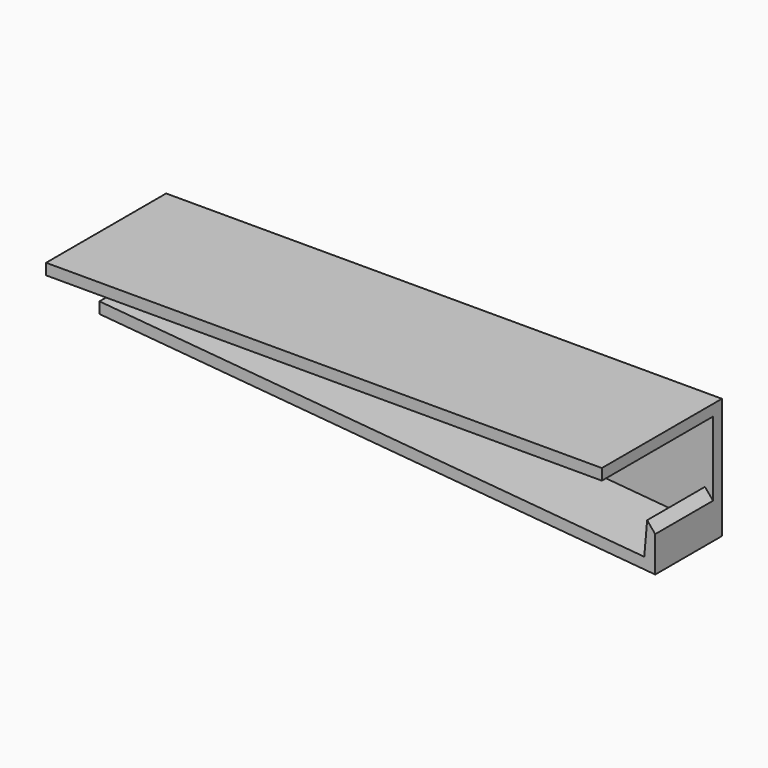
from build123d import *

# Parameters (mm, degrees)
F1_DEPTH    = 2
F3_DEPTH    = 13
F2_W        = 100
F2_H        = 2
F4_DEPTH    = 25
F5_W        = 1.9823738266
F5_H        = 13
F6_DEPTH    = 6
F7_T1_DEPTH = 18.1433659759
F9_DEPTH    = 25


# Not quite as in the source:
# - a fillet or chamfer that OpenCascade refuses, or shapes differently, is made with other operations: its cross-section is extruded or revolved along the edge and cut away or added


with BuildPart() as f1:
    # F0 (on Front) → F1 (new body)
    with BuildSketch(Plane.XZ):
        Polygon((-26.6649637938, 13), (-26.6649637938, 0), (73.3350362062, -8.7488663526), (73.3350362062, 13), align=None)
    extrude(amount=F1_DEPTH)

    # F2 (on face) → F3 (join)
    with BuildSketch(Plane.XZ.offset(2)):
        Polygon((73.3350362062, -6.7412266775), (-26.6649136147, 2.007635285), (-26.6649637938, 0), (73.3350362062, -8.7488663526), align=None)
    extrude(amount=F3_DEPTH)

    # F2 (on face) → F4 (join)
    with BuildSketch(Plane.XZ.offset(2)):
        with Locations((23.3350362062, 12)):
            Rectangle(F2_W, F2_H)
    extrude(amount=F4_DEPTH)

    # F5 (on face) → F6 (join)
    with BuildSketch(Plane(origin=(-0.0282388724, 0, -0.322771789), x_dir=(0.9961946981, 0, -0.0871557427), z_dir=(0.0871557427, 0, 0.9961946981))):
        with Locations((72.6523239577, -8.5)):
            Rectangle(F5_W, F5_H)
    extrude(amount=F6_DEPTH)

    # F7: chamfer of 2 on 1 edges, made by hand

    # F7_s2 → F7_t1 (cut)
    with BuildSketch(Plane.XZ.offset(2)):
        Polygon((73.6836591771, -2.7564478851), (71.8655812665, -0.5897470035), (73.8579706626, -0.764058489), align=None)
    extrude(amount=F7_T1_DEPTH, mode=Mode.SUBTRACT)

    # F8 (on face) → F9 (cut)
    with BuildSketch(Plane(origin=(0, -2, 0), x_dir=(-1, 0, 0), z_dir=(0, 1, 0))):
        Polygon((-73.6836591771, -2.7564478851), (-73.3350362062, -6.7412266775), (-73.3350362062, -2.340975207), align=None)
    extrude(amount=-F9_DEPTH, mode=Mode.SUBTRACT)


solid = f1.part
